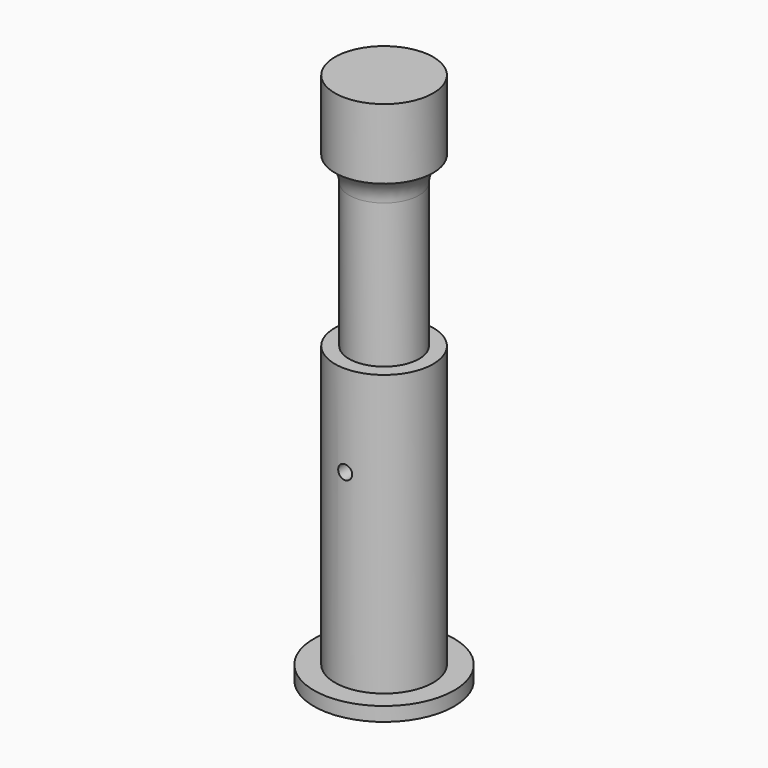
from build123d import *

# Parameters (mm, degrees)
F0_R     = 3.5
F1_DEPTH = 13
F7_R     = 3.5
F7_R_2   = 2.5
F8_DEPTH = 25
F9_START = 8
F9_DEPTH = 12
F0_R_2   = 5
F3_DEPTH = 1
F5_D     = 1
F5_DEPTH = 5.001
F6_D     = 1
F6_DEPTH = 12
F6_TIP   = 0.3004303095


# Not quite as in the source:
# - a fillet or chamfer that OpenCascade refuses, or shapes differently, is made with other operations: its cross-section is extruded or revolved along the edge and cut away or added


with BuildPart() as f1:
    # F0 (on Top) → F1 (new body)
    with BuildSketch(Plane.XY):
        Circle(F0_R)
    extrude(amount=F1_DEPTH)

    # F7 (on face) → F8 (join)
    with BuildSketch(Plane.XY.offset(13)):
        Circle(F7_R)
        Circle(F7_R_2, mode=Mode.SUBTRACT)
        Circle(F7_R_2)
    extrude(amount=F8_DEPTH)

    # F7 (on face) → F9 (cut)
    with BuildSketch(Plane.XY.offset(13).offset(F9_START)):
        Circle(F7_R)
        Circle(F7_R_2, mode=Mode.SUBTRACT)
    extrude(amount=F9_DEPTH, mode=Mode.SUBTRACT)

    # F2: fillet of radius 2 on 1 edges, made by hand

    # F2_s1 → F2_t2 (revolve)
    with BuildSketch(Plane.XZ):
        with BuildLine():
            ThreePointArc((2.5, 31.2679491924), (2.7679491924, 32.2679491924), (3.5, 33))
            Line((3.5, 33), (2.5, 33))
            Line((2.5, 33), (2.5, 31.2679491924))
        make_face()
    revolve(axis=Axis((0, 0, 33), (0, 0, 1)))

    # F0 (on Top) → F3 (join)
    with BuildSketch(Plane.XY):
        Circle(F0_R_2)
        Circle(F0_R, mode=Mode.SUBTRACT)
    extrude(amount=F3_DEPTH)

    # F5 (through all, one way)
    with BuildSketch(Plane.XZ):
        with Locations((0, 14.4967586048)):
            Circle(F5_D / 2)
    extrude(amount=-F5_DEPTH, mode=Mode.SUBTRACT)

    # F6
    with Locations(Plane(origin=(0, 0, 0), x_dir=(1, 0, 0), z_dir=(0, 1, 0))):
        with Locations((0, -14.4967586048)):
            Hole(F6_D / 2, depth=F6_DEPTH)
            with Locations((0, 0, -(F6_DEPTH + F6_TIP / 2))):  # 118° drill point
                Cone(0, F6_D / 2, F6_TIP, mode=Mode.SUBTRACT)


solid = f1.part
